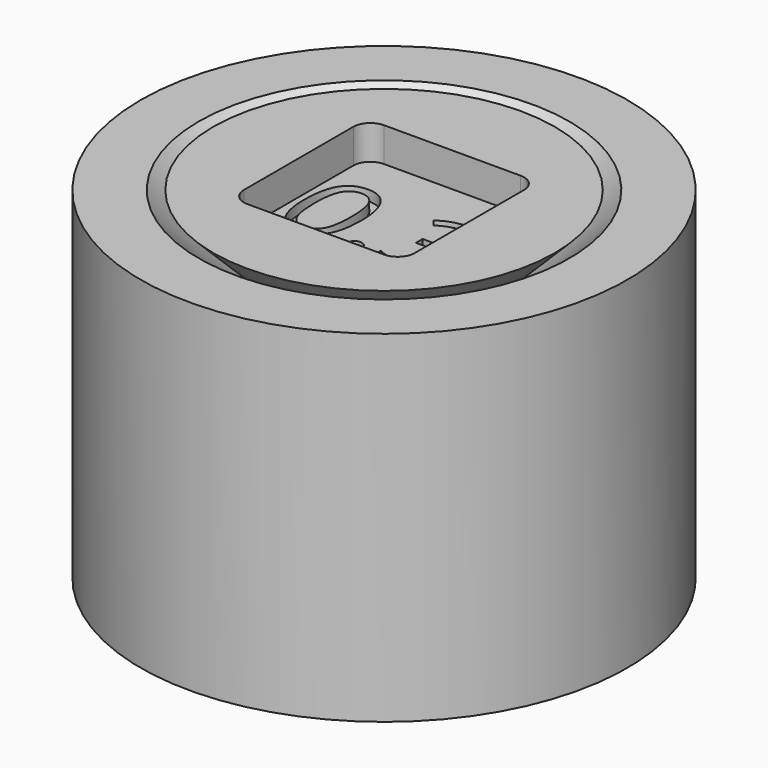
from build123d import *

# Parameters (mm, degrees)
F4_DEPTH     = 1
F5_TEXT_SIZE = 3.5316190266
F6_DEPTH     = 1.3


# Not quite as in the source:
# - Text() gives the source's letters only with a copy of the font that has no kerning and outlines rounded to 1/6400 em; it was checked with that copy


with BuildPart() as f1:
    # F0 (on Front) → F1 (revolve)
    with BuildSketch(Plane.XZ):
        with BuildLine():
            Line((-5, 0), (0, 0))
            Line((0, 0), (0, 10))
            Line((0, 10), (-5, 10))
            Line((-5, 10), (-2.7928932188, 7.7928932188))
            ThreePointArc((-2.7928932188, 7.7928932188), (-2.5761204675, 7.46846987), (-2.5, 7.0857864376))
            Line((-2.5, 7.0857864376), (-2.5, 2.9142135624))
            ThreePointArc((-2.5, 2.9142135624), (-2.5761204675, 2.53153013), (-2.7928932188, 2.2071067812))
            Line((-2.7928932188, 2.2071067812), (-5, 0))
        make_face()
    revolve(axis=Axis((0, 0, 5), (0, 0, 1)))

    # F3 (on face) → F4 (cut)
    with BuildSketch(Plane.XY.offset(10)):
        with BuildLine():
            Line((2, 2.5), (-2, 2.5))
            ThreePointArc((-2, 2.5), (-2.3535533906, 2.3535533906), (-2.5, 2))
            Line((-2.5, 2), (-2.5, -2))
            ThreePointArc((-2.5, -2), (-2.3535533906, -2.3535533906), (-2, -2.5))
            Line((-2, -2.5), (2, -2.5))
            ThreePointArc((2, -2.5), (2.3535533906, -2.3535533906), (2.5, -2))
            Line((2.5, -2), (2.5, 2))
            ThreePointArc((2.5, 2), (2.3535533906, 2.3535533906), (2, 2.5))
        make_face()
    extrude(amount=-F4_DEPTH, mode=Mode.SUBTRACT)

    # F5 (on offset) → F6 (cut)
    with BuildSketch(Plane.XY.offset(10)):
        with Locations((-2.5, -1.2713828496)):
            Text('0.3', F5_TEXT_SIZE, font='Open Sans', text_align=(TextAlign.LEFT, TextAlign.BOTTOM))
    extrude(amount=-F6_DEPTH, mode=Mode.SUBTRACT)


with BuildPart() as f1b:
    # F0 (on Front) → F1, piece 2 (revolve)
    with BuildSketch(Plane.XZ):
        with BuildLine():
            Line((-7.1242640687, 10), (-7.1242640687, 0))
            Line((-7.1242640687, 0), (-5.4242640687, 0))
            Line((-5.4242640687, 0), (-3.0928932188, 2.3313708499))
            ThreePointArc((-3.0928932188, 2.3313708499), (-2.8761204675, 2.6557941987), (-2.8, 3.0384776311))
            Line((-2.8, 3.0384776311), (-2.8, 6.9615223689))
            ThreePointArc((-2.8, 6.9615223689), (-2.8761204675, 7.3442058013), (-3.0928932188, 7.6686291501))
            Line((-3.0928932188, 7.6686291501), (-5.4242640687, 10))
            Line((-5.4242640687, 10), (-7.1242640687, 10))
        make_face()
    revolve(axis=Axis((0, 0, 5), (0, 0, 1)))


solid = Compound([f1.part, f1b.part])
